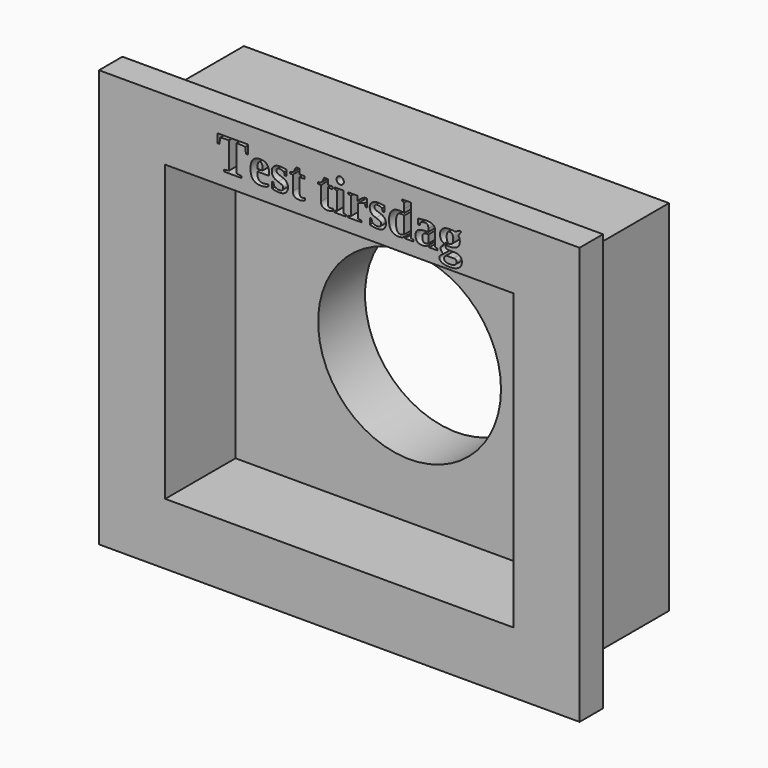
from build123d import *

# Parameters (mm, degrees)
F0_W         = 82.0367336273
F0_H         = 71.2562650442
F1_DEPTH     = 25
F2_W         = 59.4240427017
F2_H         = 50.2212010324
F3_DEPTH     = 15
F4_W         = 82.0367336273
F4_H         = 71.2562650442
F4_W_2       = 72.5709572434
F4_H_2       = 61.2646117806
F5_DEPTH     = 20
F6_R         = 15.6072164296
F7_DEPTH     = 25
F8_TEXT_SIZE = 8.251489554
F9_DEPTH     = 3


# Not quite as in the source:
# - Text() gives the source's letters only with a copy of the font that has no kerning and outlines rounded to 1/6400 em; it was checked with that copy


with BuildPart() as f1:
    # F0 (on Front) → F1 (new body)
    with BuildSketch(Plane.XZ):
        Rectangle(F0_W, F0_H)
    extrude(amount=F1_DEPTH)

    # F2 (on face) → F3 (cut)
    with BuildSketch(Plane.XZ.offset(25)):
        Rectangle(F2_W, F2_H)
    extrude(amount=-F3_DEPTH, mode=Mode.SUBTRACT)

    # F4 (on face) → F5 (cut)
    with BuildSketch(Plane(origin=(0, 0, 0), x_dir=(-1, 0, 0), z_dir=(0, 1, 0))):
        Rectangle(F4_W, F4_H)
        Rectangle(F4_W_2, F4_H_2, mode=Mode.SUBTRACT)
    extrude(amount=-F5_DEPTH, mode=Mode.SUBTRACT)

    # F6 (on face) → F7 (cut)
    with BuildSketch(Plane.XZ.offset(10)):
        Circle(F6_R)
    extrude(amount=-F7_DEPTH, mode=Mode.SUBTRACT)

    # F8 (on face) → F9 (cut)
    with BuildSketch(Plane.XZ.offset(25)):
        with Locations((-20.943091251, 27.3347180337)):
            Text('Test tirsdag', F8_TEXT_SIZE, font='Tinos', font_style=FontStyle.BOLD, text_align=(TextAlign.LEFT, TextAlign.BOTTOM))
    extrude(amount=-F9_DEPTH, mode=Mode.SUBTRACT)


solid = f1.part
